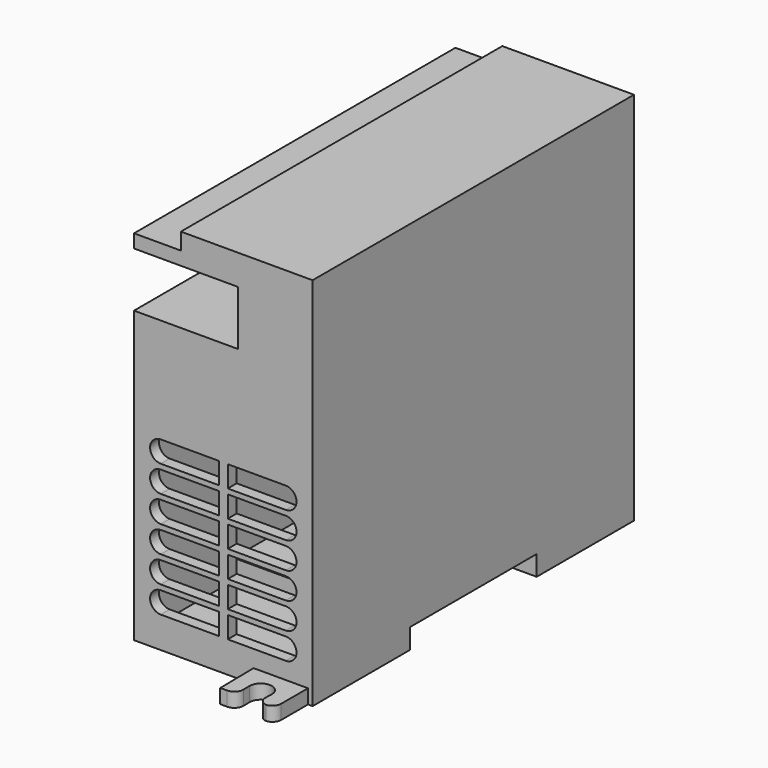
from build123d import *

# Parameters (mm, degrees)
F1_DEPTH    = 40
F3_T        = -2.5
F4_DEPTH    = 90.001
F6_DEPTH    = 90
F7_R        = 2.25
F8_DEPTH    = 3.2
F9_T1_DEPTH = 13.4224852585
F9_T3_DEPTH = 13.2


# Not quite as in the source:
# - a fillet or chamfer that OpenCascade refuses, or shapes differently, is made with other operations: its cross-section is extruded or revolved along the edge and cut away or added


with BuildPart() as f1:
    # F0 (on Right) → F1 (new body)
    with BuildSketch(Plane.YZ):
        Polygon((-45, 0), (-17.75, 0), (-17.75, 4.5), (17.75, 4.5), (17.75, 0), (45, 0), (45, 65), (-45, 65), align=None)
    extrude(amount=F1_DEPTH)

    # F3 (hollow: no face is removed)
    offset(amount=F3_T, kind=Kind.INTERSECTION, mode=Mode.SUBTRACT)

    # F2 (on face) → F4 (cut, through all)
    with BuildSketch(Plane(origin=(0, 45, 0), x_dir=(-1, 0, 0), z_dir=(0, 1, 0))):
        with BuildLine():
            Line((-21, 36.75), (-21, 41.55))
            Line((-21, 41.55), (-34, 41.55))
            ThreePointArc((-34, 41.55), (-36.4, 39.15), (-34, 36.75))
            Line((-34, 36.75), (-21, 36.75))
        make_face()
        with BuildLine():
            Line((-19, 41.55), (-19, 36.75))
            Line((-19, 36.75), (-6, 36.75))
            ThreePointArc((-6, 36.75), (-3.6, 39.15), (-6, 41.55))
            Line((-6, 41.55), (-19, 41.55))
        make_face()
        with BuildLine():
            Line((-19, 35.6), (-19, 30.8))
            Line((-19, 30.8), (-6, 30.8))
            ThreePointArc((-6, 30.8), (-3.6, 33.2), (-6, 35.6))
            Line((-6, 35.6), (-19, 35.6))
        make_face()
        with BuildLine():
            Line((-21, 30.8), (-21, 35.6))
            Line((-21, 35.6), (-34, 35.6))
            ThreePointArc((-34, 35.6), (-36.4, 33.2), (-34, 30.8))
            Line((-34, 30.8), (-21, 30.8))
        make_face()
        with BuildLine():
            Line((-21, 24.85), (-21, 29.65))
            Line((-21, 29.65), (-34, 29.65))
            ThreePointArc((-34, 29.65), (-36.4, 27.25), (-34, 24.85))
            Line((-34, 24.85), (-21, 24.85))
        make_face()
        with BuildLine():
            Line((-19, 29.65), (-19, 24.85))
            Line((-19, 24.85), (-6, 24.85))
            ThreePointArc((-6, 24.85), (-3.6, 27.25), (-6, 29.65))
            Line((-6, 29.65), (-19, 29.65))
        make_face()
        with BuildLine():
            Line((-21, 18.9), (-21, 23.7))
            Line((-21, 23.7), (-34, 23.7))
            ThreePointArc((-34, 23.7), (-36.4, 21.3), (-34, 18.9))
            Line((-34, 18.9), (-21, 18.9))
        make_face()
        with BuildLine():
            Line((-19, 23.7), (-19, 18.9))
            Line((-19, 18.9), (-6, 18.9))
            ThreePointArc((-6, 18.9), (-3.6, 21.3), (-6, 23.7))
            Line((-6, 23.7), (-19, 23.7))
        make_face()
        with BuildLine():
            Line((-21, 12.95), (-21, 17.75))
            Line((-21, 17.75), (-34, 17.75))
            ThreePointArc((-34, 17.75), (-36.4, 15.35), (-34, 12.95))
            Line((-34, 12.95), (-21, 12.95))
        make_face()
        with BuildLine():
            Line((-19, 17.75), (-19, 12.95))
            Line((-19, 12.95), (-6, 12.95))
            ThreePointArc((-6, 12.95), (-3.6, 15.35), (-6, 17.75))
            Line((-6, 17.75), (-19, 17.75))
        make_face()
        with BuildLine():
            Line((-34, 7), (-21, 7))
            Line((-21, 7), (-21, 11.8))
            Line((-21, 11.8), (-34, 11.8))
            ThreePointArc((-34, 11.8), (-36.4, 9.4), (-34, 7))
        make_face()
        with BuildLine():
            Line((-19, 11.8), (-19, 7))
            Line((-19, 7), (-6, 7))
            ThreePointArc((-6, 7), (-3.6, 9.4), (-6, 11.8))
            Line((-6, 11.8), (-19, 11.8))
        make_face()
    extrude(amount=-F4_DEPTH, mode=Mode.SUBTRACT)

    # F5 (on face) → F6 (join)
    with BuildSketch(Plane.XZ.offset(45)):
        Polygon((23.3, 65), (40, 65), (40, 84), (10.5, 84), (10.5, 80.25), (0, 80.25), (0, 77.25), (23.3, 77.25), align=None)
    extrude(amount=-F6_DEPTH)


with BuildPart() as f8:
    # F7 (on Top) → F8 (new body)
    with BuildSketch(Plane.XY):
        with BuildLine():
            Line((0, 50.0000204146), (0, 45.0000204146))
            Line((0, 45.0000204146), (13, 45.0000204146))
            Line((13, 45.0000204146), (13, 50.0000204146))
            ThreePointArc((13, 50.0000204146), (6.5, 56.5000204146), (0, 50.0000204146))
        make_face()
        with Locations((6.5, 51.9500204146)):
            Circle(F7_R, mode=Mode.SUBTRACT)
    extrude(amount=F8_DEPTH)


with BuildPart() as f8b:
    # F7 (on Top) → F8, piece 2 (new body)
    with BuildSketch(Plane.XY):
        with BuildLine():
            Line((38.9799938861, -54.5024834573), (38.9799938861, -45.0004808827))
            Line((38.9799938861, -45.0004808827), (26.7799938861, -45.0004808827))
            Line((26.7799938861, -45.0004808827), (26.9155632704, -54.5024834573))
            Line((26.9155632704, -54.5024834573), (30.5308417415, -54.5024834573))
            Line((30.5308417415, -54.5024834573), (30.4483837113, -50.755483601))
            ThreePointArc((30.4483837113, -50.755483601), (32.9202755548, -48.2006321706), (35.4477785783, -50.7004808827))
            ThreePointArc((35.4477785783, -50.7004808827), (35.4476272904, -50.7279839062), (35.4471734452, -50.755483601))
            Line((35.4471734452, -50.755483601), (35.364715415, -54.5024834573))
            Line((35.364715415, -54.5024834573), (38.9799938861, -54.5024834573))
        make_face()
    extrude(amount=F8_DEPTH)

    # F9: fillet of radius 2 on 3 edges, made by hand

    # F9_s2 → F9_t1 (cut)
    with BuildSketch(Plane.XY.offset(-5.1112426292)):
        with BuildLine():
            ThreePointArc((28.4863446898, -54.5024834573), (29.9160307304, -53.9010533789), (30.4858605834, -52.4584812827))
            Line((30.4858605834, -52.4584812827), (30.5308417415, -54.5024834573))
            Line((30.5308417415, -54.5024834573), (28.4863446898, -54.5024834573))
        make_face()
        with BuildLine():
            ThreePointArc((35.4096965732, -52.4584812827), (35.9795264262, -53.9010533789), (37.4092124667, -54.5024834573))
            Line((37.4092124667, -54.5024834573), (35.364715415, -54.5024834573))
            Line((35.364715415, -54.5024834573), (35.4096965732, -52.4584812827))
        make_face()
    extrude(amount=F9_T1_DEPTH, mode=Mode.SUBTRACT)

    # F9_s4 → F9_t3 (cut)
    with BuildSketch(Plane.XY.offset(-5)):
        with BuildLine():
            ThreePointArc((36.9799938861, -54.5024834573), (38.3942074485, -53.9166970197), (38.9799938861, -52.5024834573))
            Line((38.9799938861, -52.5024834573), (38.9799938861, -54.5024834573))
            Line((38.9799938861, -54.5024834573), (36.9799938861, -54.5024834573))
        make_face()
    extrude(amount=F9_T3_DEPTH, mode=Mode.SUBTRACT)


solid = Compound([f1.part, f8.part, f8b.part])
